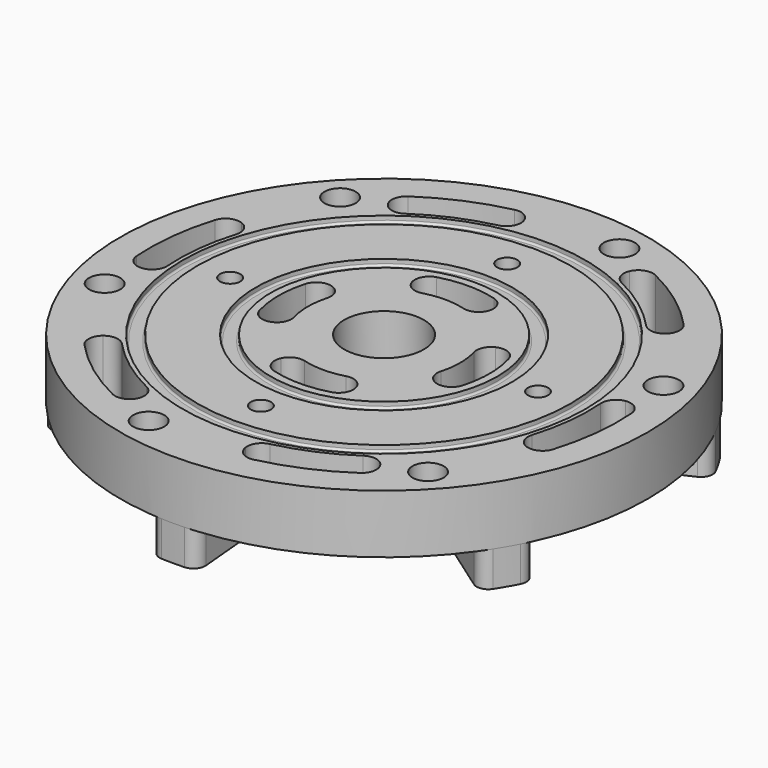
from build123d import *

# Parameters (mm, degrees)
F0_R             = 57.15
F1_DEPTH         = 12.7
F2_R             = 8.636
F3_DEPTH         = 12.701
F5_DEPTH         = 7.62
F6_T1_DEPTH      = 14.2671475518
F6_T3_DEPTH      = 13.7344913133
F8_COUNT         = 6
F9_D             = 4.3942
F9_DEPTH         = 15.24
F9_TIP           = 1.3201508661
F10_R            = 43.6245
F10_R_2          = 40.4241
F11_DEPTH        = 1.2954
F12_R            = 0.4064
F14_DEPTH        = 20.321
F14_COPIES_COUNT = 6
F15_R            = 3.17499
F16_R            = 27.7495
F16_R_2          = 24.5491
F17_DEPTH        = 1.2954
F18_R            = 0.4064
F20_DEPTH        = 20.321
F20_COPIES_COUNT = 4
F21_R            = 3.17499
F23_D            = 4.3942
F23_DEPTH        = 6.35
F23_TIP          = 1.3201508661
F25_D            = 6.7564


# Not quite as in the source:
# - a fillet or chamfer that OpenCascade refuses, or shapes differently, is made with other operations: its cross-section is extruded or revolved along the edge and cut away or added
# - a fillet or chamfer is up to 0.001 mm smaller than in the source, because OpenCascade refuses the exact size
# - a pattern or mirror of a feature is missing from the dataset's text; its kind, count and spacing are read off the source's solid


with BuildPart() as f1:
    # F0 (on Top) → F1 (new body)
    with BuildSketch(Plane.XY):
        Circle(F0_R)
    extrude(amount=F1_DEPTH)

    # F2 (on face) → F3 (cut, through all)
    with BuildSketch(Plane.XY.offset(12.7)):
        Circle(F2_R)
    extrude(amount=-F3_DEPTH, mode=Mode.SUBTRACT)

    # F4 (on face) → F5 (join)
    with BuildSketch(Plane(origin=(0, 0, 0), x_dir=(1, 0, 0), z_dir=(0, 0, -1))):
        with BuildLine():
            Line((-2.8575, -31.6211510504), (-5.1435, -56.9180718907))
            ThreePointArc((-5.1435, -56.9180718907), (0, -57.15), (5.1435, -56.9180718907))
            Line((5.1435, -56.9180718907), (2.8575, -31.6211510504))
            ThreePointArc((2.8575, -31.6211510504), (0, -31.75), (-2.8575, -31.6211510504))
        make_face()
    extrude(amount=F5_DEPTH)

    # F6: fillet of radius 2.54 on 4 edges, made by hand

    # F6_s2 → F6_t1 (cut)
    with BuildSketch(Plane.XY.offset(-14.2671475518)):
        with BuildLine():
            ThreePointArc((2.490581259, 57.0957047858), (4.2919178251, 56.2301660065), (4.9095808426, 54.3295179065))
            Line((4.9095808426, 54.3295179065), (5.1435, 56.9180718907))
            ThreePointArc((5.1435, 56.9180718907), (3.8180737982, 57.022318547), (2.490581259, 57.0957047858))
        make_face()
        with BuildLine():
            ThreePointArc((-2.490581259, 57.0957047858), (-4.2919178251, 56.2301660065), (-4.9095808426, 54.3295179065))
            Line((-4.9095808426, 54.3295179065), (-5.1435, 56.9180718907))
            ThreePointArc((-5.1435, 56.9180718907), (-3.8180737982, 57.022318547), (-2.490581259, 57.0957047858))
        make_face()
    extrude(amount=F6_T1_DEPTH, mode=Mode.SUBTRACT)

    # F6_s4 → F6_t3 (cut)
    with BuildSketch(Plane.XY.offset(-13.7344913133)):
        with BuildLine():
            ThreePointArc((0.5073422252, 31.7459462588), (2.2462164703, 32.396860006), (3.0776216873, 34.0570219595))
            Line((3.0776216873, 34.0570219595), (2.8575, 31.6211510504))
            ThreePointArc((2.8575, 31.6211510504), (1.6835778156, 31.7053318188), (0.5073422252, 31.7459462588))
        make_face()
        with BuildLine():
            ThreePointArc((-3.0776216873, 34.0570219595), (-2.2462164703, 32.396860006), (-0.5073422252, 31.7459462588))
            ThreePointArc((-0.5073422252, 31.7459462588), (-1.6835778156, 31.7053318188), (-2.8575, 31.6211510504))
            Line((-2.8575, 31.6211510504), (-3.0776216873, 34.0570219595))
        make_face()
    extrude(amount=F6_T3_DEPTH, mode=Mode.SUBTRACT)

    # F8: F1 ×6 about axis
    f8_axis = Axis((0, 0, 12.7), (0, 0, 1))


with BuildPart() as f1_1:
    add(f1.part)
    for i in range(1, F8_COUNT):
        add(f1.part.rotate(f8_axis, i * 360 / F8_COUNT))

    # F9
    with Locations(Plane(origin=(0, 0, -7.62), x_dir=(1, 0, 0), z_dir=(0, 0, -1))):
        with Locations((0, -50.8), (43.9940905122, -25.4), (43.9940905122, 25.4), (0, 50.8), (-43.9940905122, 25.4), (-43.9940905122, -25.4)):
            Hole(F9_D / 2, depth=F9_DEPTH)
            with Locations((0, 0, -(F9_DEPTH + F9_TIP / 2))):  # 118° drill point
                Cone(0, F9_D / 2, F9_TIP, mode=Mode.SUBTRACT)

    # F10 (on face) → F11 (cut)
    with BuildSketch(Plane.XY.offset(12.7)):
        Circle(F10_R)
        Circle(F10_R_2, mode=Mode.SUBTRACT)
    extrude(amount=-F11_DEPTH, mode=Mode.SUBTRACT)

    # F12
    f12_edges = [f1_1.edges().sort_by_distance(p)[0] for p in [
        (-43.6245, 0, 11.4046),
        (-40.4241, 0, 11.4046),
    ]]
    fillet(f12_edges, radius=F12_R)

    # F13 (on face) → F14 (cut, through all)
    with BuildSketch(Plane.XY.offset(12.7)):
        with BuildLine():
            ThreePointArc((16.721010174, 41.1850739803), (26.4387827868, 35.7322440487), (34.49502146, 28.0338365993))
            Line((34.49502146, 28.0338365993), (39.4228816685, 32.0386703992))
            ThreePointArc((39.4228816685, 32.0386703992), (30.2157517563, 40.8368503413), (19.1097259131, 47.0686559775))
            Line((19.1097259131, 47.0686559775), (16.721010174, 41.1850739803))
        make_face()
    f14 = extrude(amount=-F14_DEPTH, mode=Mode.SUBTRACT)

    # F14_copies: F14 ×6 about axis
    f14_copies_axis = Axis((0, 0, 0), (0, 0, 1))
    for i in range(1, F14_COPIES_COUNT):
        add(f14.rotate(f14_copies_axis, i * 360 / F14_COPIES_COUNT), mode=Mode.SUBTRACT)

    # F15 (radius 3.175 in the source; OpenCascade refuses exactly that, so slightly less here)
    f15_edges = [f1_1.edges().sort_by_distance(p)[0] for p in [
        (39.422882, 32.03867, 6.35),
        (19.109726, 47.068656, 6.35),
        (16.72101, 41.185074, 6.35),
        (34.495021, 28.033837, 6.35),
    ]]
    fillet(f15_edges, radius=F15_R)

    # F16 (on face) → F17 (cut)
    with BuildSketch(Plane.XY.offset(12.7)):
        Circle(F16_R)
        Circle(F16_R_2, mode=Mode.SUBTRACT)
    extrude(amount=-F17_DEPTH, mode=Mode.SUBTRACT)

    # F18
    f18_edges = [f1_1.edges().sort_by_distance(p)[0] for p in [
        (-27.7495, 0, 11.4046),
        (-24.5491, 0, 11.4046),
    ]]
    fillet(f18_edges, radius=F18_R)

    # F19 (on face) → F20 (cut, through all)
    with BuildSketch(Plane.XY.offset(12.7)):
        with BuildLine():
            Line((9.6610534634, -20.7181960117), (6.9774275013, -14.963141564))
            ThreePointArc((6.9774275013, -14.963141564), (0, -16.51), (-6.9774275013, -14.963141564))
            Line((-6.9774275013, -14.963141564), (-9.6610534634, -20.7181960117))
            ThreePointArc((-9.6610534634, -20.7181960117), (0, -22.86), (9.6610534634, -20.7181960117))
        make_face()
    f20 = extrude(amount=-F20_DEPTH, mode=Mode.SUBTRACT)

    # F20_copies: F20 ×4 about axis
    f20_copies_axis = Axis((0, 0, 0), (0, 0, 1))
    for i in range(1, F20_COPIES_COUNT):
        add(f20.rotate(f20_copies_axis, i * 360 / F20_COPIES_COUNT), mode=Mode.SUBTRACT)

    # F21 (radius 3.175 in the source; OpenCascade refuses exactly that, so slightly less here)
    f21_edges = [f1_1.edges().sort_by_distance(p)[0] for p in [
        (-6.977428, -14.963142, 6.35),
        (-9.661053, -20.718196, 6.35),
        (6.977428, -14.963142, 6.35),
        (9.661053, -20.718196, 6.35),
        (14.963142, 6.977428, 6.35),
        (20.718196, 9.661053, 6.35),
        (20.718196, -9.661053, 6.35),
        (14.963142, -6.977428, 6.35),
        (-14.963142, -6.977428, 6.35),
        (-20.718196, -9.661053, 6.35),
        (-14.963142, 6.977428, 6.35),
        (-20.718196, 9.661053, 6.35),
        (-6.977428, 14.963142, 6.35),
        (-9.661053, 20.718196, 6.35),
        (9.661053, 20.718196, 6.35),
        (6.977428, 14.963142, 6.35),
        (-16.72101, -41.185074, 6.35),
        (-19.109726, -47.068656, 6.35),
        (-39.422882, -32.03867, 6.35),
        (-34.495021, -28.033837, 6.35),
        (27.306815, -35.073357, 6.35),
        (31.207789, -40.083836, 6.35),
        (8.034862, -50.160552, 6.35),
        (7.030504, -43.890483, 6.35),
        (44.027825, 6.111717, 6.35),
        (50.317515, 6.98482, 6.35),
        (47.457743, -18.121882, 6.35),
        (41.525525, -15.856647, 6.35),
        (-44.027825, -6.111717, 6.35),
        (-50.317515, -6.98482, 6.35),
        (-47.457743, 18.121882, 6.35),
        (-41.525525, 15.856647, 6.35),
        (-27.306815, 35.073357, 6.35),
        (-31.207789, 40.083836, 6.35),
        (-8.034862, 50.160552, 6.35),
        (-7.030504, 43.890483, 6.35),
    ]]
    fillet(f21_edges, radius=F21_R)

    # F23
    with Locations(Plane.XY.offset(12.7)):
        with Locations((-33.3375, 0), (0, -33.3375), (33.3375, 0), (0, 33.3375)):
            Hole(F23_D / 2, depth=F23_DEPTH)
            with Locations((0, 0, -(F23_DEPTH + F23_TIP / 2))):  # 118° drill point
                Cone(0, F23_D / 2, F23_TIP, mode=Mode.SUBTRACT)

    # F25 (through all)
    with Locations(Plane.XY.offset(12.7)):
        with Locations((11.3576544358, 49.5140756323), (48.5592745603, 14.9210205473), (37.2016201245, -34.593055085), (-11.3576544358, -49.5140756323), (-48.5592745603, -14.9210205473), (-37.2016201245, 34.593055085)):
            Hole(F25_D / 2)


solid = f1_1.part
